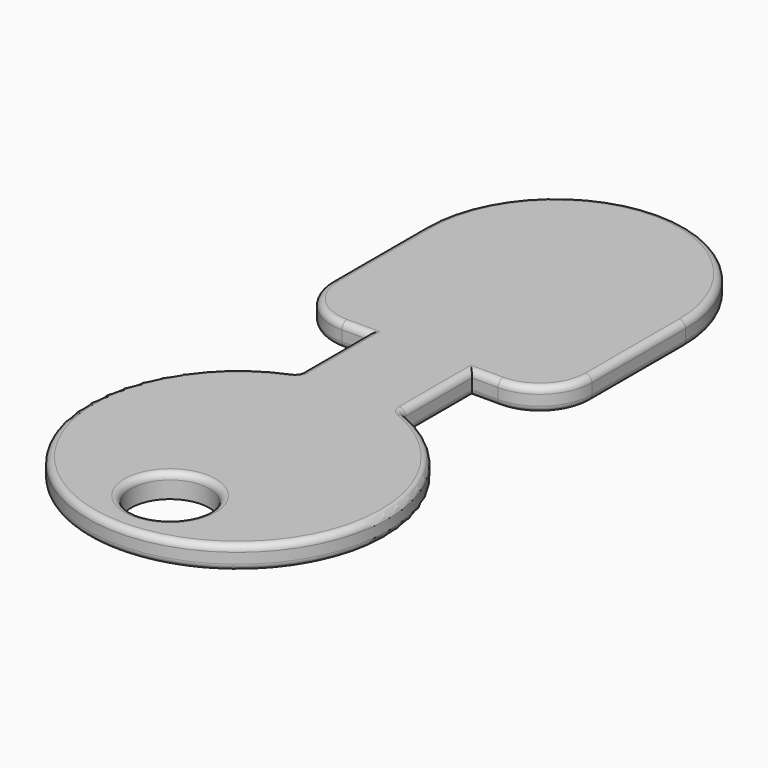
from build123d import *

# Parameters (mm, degrees)
F0_R     = 3
F1_DEPTH = 1.8
F2_R     = 4
F3_R     = 4
F4_R     = 0.5


with BuildPart() as f1:
    # F0 (on Top) → F1 (new body)
    with BuildSketch(Plane.XY):
        with BuildLine():
            Line((-4, 17.5), (-4, 10.7819293264))
            ThreePointArc((-4, 10.7819293264), (0, -11.5), (4, 10.7819293264))
            Line((4, 10.7819293264), (4, 17.5))
            Line((4, 17.5), (10, 17.5))
            Line((10, 17.5), (10, 30.5))
            ThreePointArc((10, 30.5), (0, 40.5), (-10, 30.5))
            Line((-10, 30.5), (-10, 17.5))
            Line((-10, 17.5), (-4, 17.5))
        make_face()
        with Locations((0, -6.5)):
            Circle(F0_R, mode=Mode.SUBTRACT)
    extrude(amount=F1_DEPTH)

    # F2
    f2_edges = [f1.edges().sort_by_distance(p)[0] for p in [
        (10, 17.5, 0.9),
    ]]
    fillet(f2_edges, radius=F2_R)

    # F3
    f3_edges = [f1.edges().sort_by_distance(p)[0] for p in [
        (-10, 17.5, 0.9),
    ]]
    fillet(f3_edges, radius=F3_R)

    # F4
    f4_edges = [f1.edges().sort_by_distance(p)[0] for p in [
        (-10, 26, 1.8),
        (-8.828427, 18.671573, 1.8),
        (0, 40.5, 1.8),
        (-5, 17.5, 1.8),
        (10, 26, 1.8),
        (-4, 14.140965, 1.8),
        (8.828427, 18.671573, 1.8),
        (0, -11.5, 1.8),
        (5, 17.5, 1.8),
        (4, 14.140965, 1.8),
        (-3, -6.5, 1.8),
        (-4, 10.781929, 0.9),
        (4, 10.781929, 0.9),
        (0, -11.5, 0),
        (10, 26, 0),
        (8.828427, 18.671573, 0),
        (5, 17.5, 0),
        (-10, 26, 0),
        (-8.828427, 18.671573, 0),
        (0, 40.5, 0),
        (-5, 17.5, 0),
        (-4, 14.140965, 0),
        (4, 14.140965, 0),
    ]]
    fillet(f4_edges, radius=F4_R)


solid = f1.part
